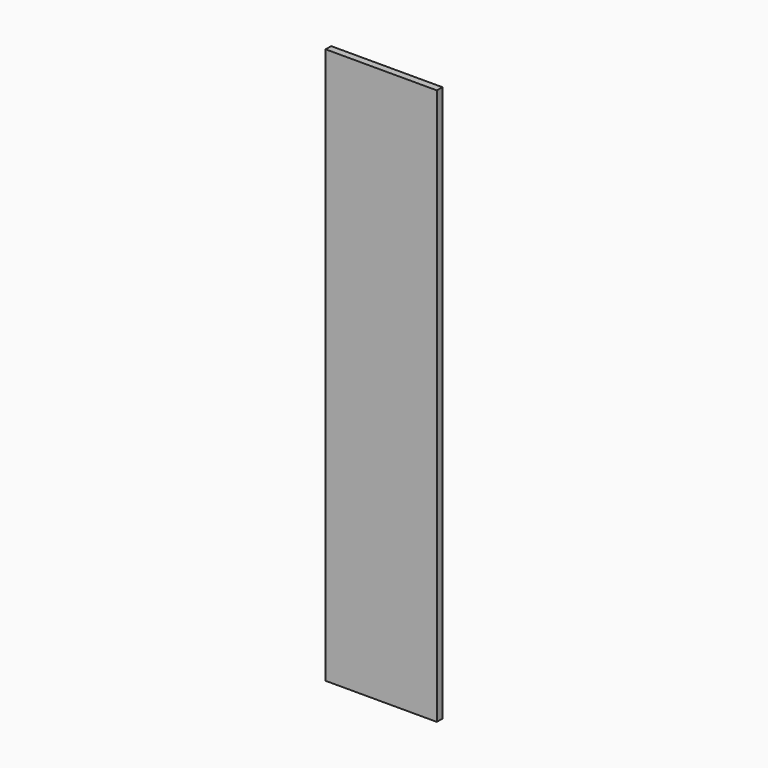
from build123d import *

# Parameters (mm, degrees)
F0_W     = 50.8
F0_H     = 253.87046
F1_DEPTH = 3.175


# Not quite as in the source:
# - a length typed as a fraction of an inch, garbled in the dataset ("3 / 203.2 mm" for 3/8 in), is restored


with BuildPart() as f1:
    # F0 (on Front) → F1 (new body)
    with BuildSketch(Plane.XZ):
        Rectangle(F0_W, F0_H)
    extrude(amount=F1_DEPTH)


solid = f1.part
